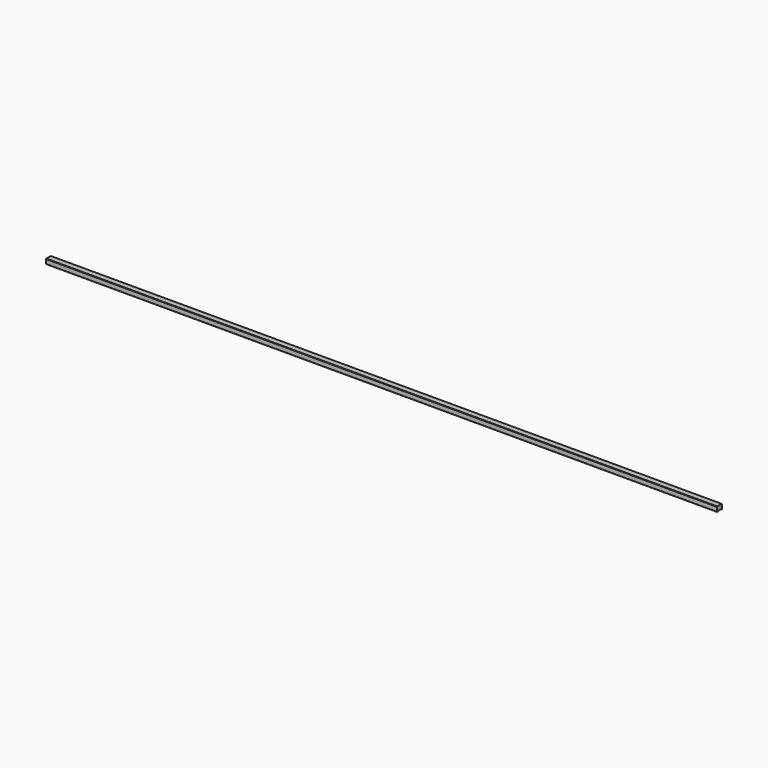
from build123d import *

# Parameters (mm, degrees)
F1_DEPTH = 10840
F2_SIZE  = 5


# Not quite as in the source:
# - a feature names something its author has since deleted; it is built from what else it names


with BuildPart() as f1:
    # F0 (on Right) → F1 (new body)
    with BuildSketch(Plane.YZ):
        Polygon((-15, 0), (0, 0), (0, 80), (-100, 80), (-100, 0), (-85, 0), (-85, 8), (-15, 8), align=None)
    extrude(amount=F1_DEPTH)

    # F2
    f2_edges = [f1.edges().sort_by_distance(p)[0] for p in [
        (5420, -100, 0),
        (5420, -100, 80),
        (5420, 0, 80),
        (5420, 0, 0),
        (5420, -15, 0),
        (5420, -85, 0),
    ]]
    chamfer(f2_edges, length=F2_SIZE)


solid = f1.part
